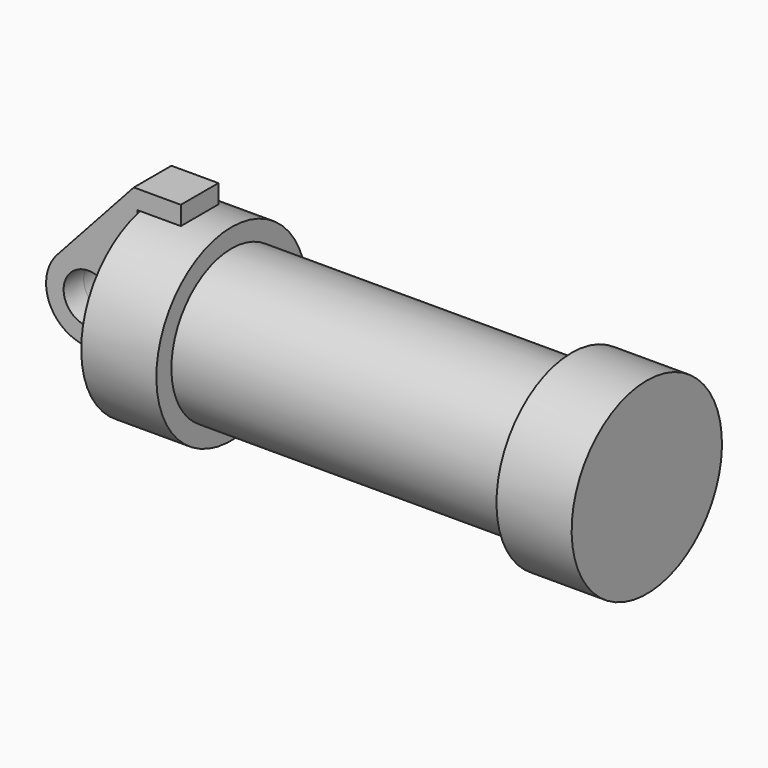
from build123d import *

# Parameters (mm, degrees)
F0_R          = 3.175
F1_DEPTH      = 3.175
F1_DEPTH_BACK = 3.175
F2_DEPTH      = 3.176
F2_TAPER      = -3
F2_DEPTH_BACK = 3.176
F0_W          = 5.842
F0_H          = 12.7


with BuildPart() as f1:
    # F0 (on Front) → F1 (new body, two sides)
    with BuildSketch(Plane.XZ) as f1_sk:
        with BuildLine():
            Line((-0.9398, 0), (0, 0))
            Line((0, 0), (0, 12.7))
            Line((0, 12.7), (5.842, 12.7))
            Line((5.842, 12.7), (5.842, 15.24))
            Line((5.842, 15.24), (-0.508, 15.24))
            Line((-0.508, 15.24), (-10.8806298187, 3.8475430269))
            ThreePointArc((-10.8806298187, 3.8475430269), (-4.5919612295, 5.3297205562), (-0.9398, 0))
        make_face()
        with BuildLine():
            Line((5.842, 0), (0, 0))
            Line((0, 0), (-0.9398, 0))
            ThreePointArc((-0.9398, 0), (-3.1957909266, -4.5493385486), (-8.1826630726, -5.5069827884))
            Line((-8.1826630726, -5.5069827884), (5.842, -9.398))
            Line((5.842, -9.398), (5.842, 0))
        make_face()
        with BuildLine():
            ThreePointArc((-8.1826630726, -5.5069827884), (-3.1957909266, -4.5493385486), (-0.9398, 0))
            ThreePointArc((-0.9398, 0), (-4.5919612295, 5.3297205562), (-10.8806298187, 3.8475430269))
            ThreePointArc((-10.8806298187, 3.8475430269), (-12.1459778134, -1.5837270034), (-8.1826630726, -5.5069827884))
        make_face()
        with Locations((-6.6548, 0)):
            Circle(F0_R, mode=Mode.SUBTRACT)
        with Locations((-6.6548, 0)):
            Circle(F0_R)
    extrude(amount=F1_DEPTH)
    extrude(f1_sk.sketch, amount=-F1_DEPTH_BACK)

    # F0 (on Front) → F2 (cut, two sides)
    with BuildSketch(Plane.XZ) as f2_sk:
        with Locations((-6.6548, 0)):
            Circle(F0_R)
    extrude(amount=F2_DEPTH, taper=F2_TAPER, mode=Mode.SUBTRACT)
    extrude(f2_sk.sketch, amount=-F2_DEPTH_BACK, mode=Mode.SUBTRACT)


with BuildPart() as f3:
    # F0 (on Front) → F3 (revolve)
    with BuildSketch(Plane.XZ):
        with Locations((2.921, 6.35)):
            Rectangle(F0_W, F0_H)
        Polygon((5.842, 12.7), (5.842, 0), (66.294, 0), (66.294, 12.7), (56.134, 12.7), (56.134, 10.16), (10.16, 10.16), (10.16, 12.7), align=None)
    revolve(axis=Axis((33.147, 0, 0), (-1, 0, 0)))


solid = Compound([f1.part, f3.part])
